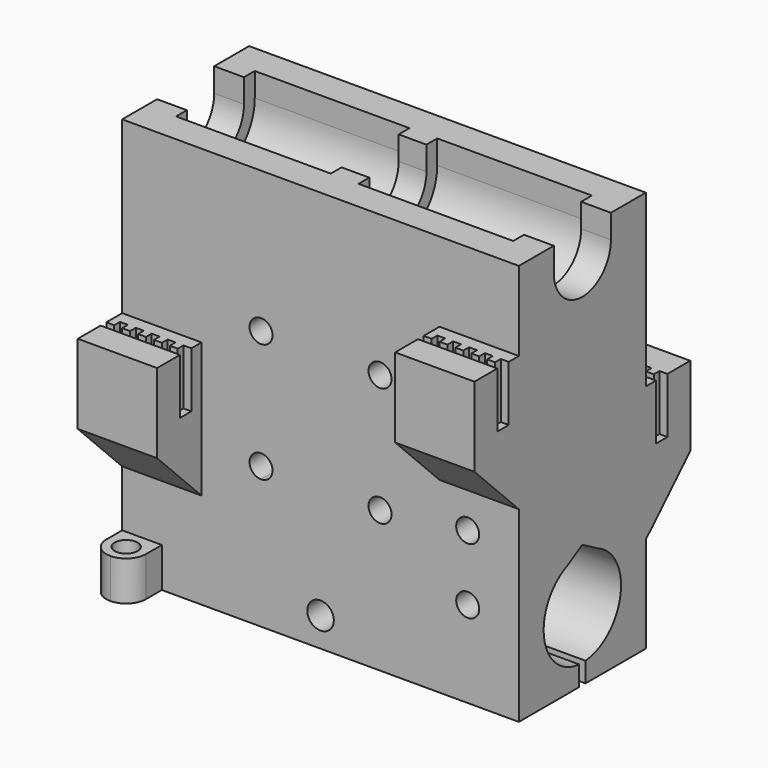
from build123d import *

# Parameters (mm, degrees)
F0_W         = 50
F0_H         = 20
F1_DEPTH     = 50.6
F3_DEPTH     = 50.001
F4_DEPTH     = 46.25
F5_DEPTH     = 26.75
F6_DEPTH     = 23.25
F7_DEPTH     = 3.75
F8_W         = 10
F8_H         = 20
F9_DEPTH     = 7
F10_T4_DEPTH = 61.4336597593
F10_T9_DEPTH = 61.4336597593
F12_DEPTH    = 7
F14_DEPTH    = 7
F15_W        = 10
F15_H        = 20
F16_DEPTH    = 7
F18_DEPTH    = 7
F20_DEPTH    = 7
F21_T4_DEPTH = 61.4336597593
F21_T9_DEPTH = 61.4336597593
F22_R        = 1.45
F22_R_2      = 1.675
F23_DEPTH    = 27.001
F24_R        = 1.45
F25_DEPTH    = 5
F26_W        = 5
F26_H        = 5
F27_DEPTH    = 5
F29_DEPTH    = 25
F30_R        = 2.49999
F32_DEPTH    = 4.5


# Not quite as in the source:
# - a fillet or chamfer that OpenCascade refuses, or shapes differently, is made with other operations: its cross-section is extruded or revolved along the edge and cut away or added
# - a fillet or chamfer is up to 0.001 mm smaller than in the source, because OpenCascade refuses the exact size


with BuildPart() as f1:
    # F0 (on Top) → F1 (new body)
    with BuildSketch(Plane.XY):
        with Locations((25, 10)):
            Rectangle(F0_W, F0_H)
    extrude(amount=F1_DEPTH)

    # F2 (on face) → F3 (cut, through all)
    with BuildSketch(Plane(origin=(0, 0, 0), x_dir=(0, -1, 0), z_dir=(-1, 0, 0))):
        with BuildLine():
            Line((-7.5528932501, 14.1876353276), (-6.3860941653, 13.5142328616))
            ThreePointArc((-6.3860941653, 13.5142328616), (-6.9508466572, 13.8832436904), (-7.5528932501, 14.1876353276))
        make_face()
        with BuildLine():
            ThreePointArc((-12.4471067499, 14.1876353276), (-13.0491533428, 13.8832436904), (-13.6139058347, 13.5142328616))
            Line((-13.6139058347, 13.5142328616), (-12.4471067499, 14.1876353276))
        make_face()
        with BuildLine():
            Line((-9.5, 0), (-9.5, 2.5205263386))
            ThreePointArc((-9.5, 2.5205263386), (-10, 2.5), (-10.5, 2.5205263386))
            Line((-10.5, 2.5205263386), (-10.5, 0))
            Line((-10.5, 0), (-10, 0))
            Line((-10, 0), (-9.5, 0))
        make_face()
        with BuildLine():
            ThreePointArc((-10.5, 2.5205263386), (-10, 2.5), (-9.5, 2.5205263386))
            Line((-9.5, 2.5205263386), (-10.5, 2.5205263386))
        make_face()
        with BuildLine():
            ThreePointArc((-10, 14.7), (-8.7499151026, 14.5705349634), (-7.5528932501, 14.1876353276))
            Line((-7.5528932501, 14.1876353276), (-10, 15.5999502167))
            Line((-10, 15.5999502167), (-10, 14.7))
        make_face()
        with BuildLine():
            ThreePointArc((-12.4471067499, 14.1876353276), (-11.2500848974, 14.5705349634), (-10, 14.7))
            Line((-10, 14.7), (-10, 15.5999502167))
            Line((-10, 15.5999502167), (-12.4471067499, 14.1876353276))
        make_face()
        with BuildLine():
            ThreePointArc((-9.5, 2.5205263386), (-5.5133531452, 4.467204336), (-3.9, 8.6))
            ThreePointArc((-3.9, 8.6), (-4.5568930935, 11.3536497969), (-6.3860941653, 13.5142328616))
            Line((-6.3860941653, 13.5142328616), (-7.5528932501, 14.1876353276))
            ThreePointArc((-7.5528932501, 14.1876353276), (-8.7499151026, 14.5705349634), (-10, 14.7))
            ThreePointArc((-10, 14.7), (-11.2500848974, 14.5705349634), (-12.4471067499, 14.1876353276))
            Line((-12.4471067499, 14.1876353276), (-13.6139058347, 13.5142328616))
            ThreePointArc((-13.6139058347, 13.5142328616), (-15.8691099055, 6.937607472), (-10.5, 2.5205263386))
            Line((-10.5, 2.5205263386), (-9.5, 2.5205263386))
        make_face()
        with BuildLine():
            Line((-5.5, 47.6), (-5.5, 50.6))
            Line((-5.5, 50.6), (-6.6458980338, 50.6))
            ThreePointArc((-6.6458980338, 50.6), (-5.7962243847, 49.205699404), (-5.5, 47.6))
        make_face()
        with BuildLine():
            Line((-13.3541019662, 50.6), (-14.5, 50.6))
            Line((-14.5, 50.6), (-14.5, 47.6))
            ThreePointArc((-14.5, 47.6), (-14.2037756153, 49.205699404), (-13.3541019662, 50.6))
        make_face()
        with BuildLine():
            ThreePointArc((-14.5, 47.6), (-10, 43.1), (-5.5, 47.6))
            ThreePointArc((-5.5, 47.6), (-5.7962243847, 49.205699404), (-6.6458980338, 50.6))
            Line((-6.6458980338, 50.6), (-13.3541019662, 50.6))
            ThreePointArc((-13.3541019662, 50.6), (-14.2037756153, 49.205699404), (-14.5, 47.6))
        make_face()
    extrude(amount=-F3_DEPTH, mode=Mode.SUBTRACT)

    # F2 (on face) → F4 (cut)
    with BuildSketch(Plane(origin=(0, 0, 0), x_dir=(0, -1, 0), z_dir=(-1, 0, 0))):
        with BuildLine():
            ThreePointArc((-16.2, 47.6), (-10, 41.4), (-3.8, 47.6))
            ThreePointArc((-3.8, 47.6), (-3.9966527372, 49.1491357726), (-4.5741360135, 50.6))
            Line((-4.5741360135, 50.6), (-5.5, 50.6))
            Line((-5.5, 50.6), (-5.5, 47.6))
            ThreePointArc((-5.5, 47.6), (-10, 43.1), (-14.5, 47.6))
            Line((-14.5, 47.6), (-14.5, 50.6))
            Line((-14.5, 50.6), (-15.4258639865, 50.6))
            ThreePointArc((-15.4258639865, 50.6), (-16.0033472628, 49.1491357726), (-16.2, 47.6))
        make_face()
        with BuildLine():
            Line((-15.4258639865, 50.6), (-16.2, 50.6))
            Line((-16.2, 50.6), (-16.2, 47.6))
            ThreePointArc((-16.2, 47.6), (-16.0033472628, 49.1491357726), (-15.4258639865, 50.6))
        make_face()
        with BuildLine():
            Line((-3.8, 47.6), (-3.8, 50.6))
            Line((-3.8, 50.6), (-4.5741360135, 50.6))
            ThreePointArc((-4.5741360135, 50.6), (-3.9966527372, 49.1491357726), (-3.8, 47.6))
        make_face()
    extrude(amount=-F4_DEPTH, mode=Mode.SUBTRACT)

    # F2 (on face) → F5 (join)
    with BuildSketch(Plane(origin=(0, 0, 0), x_dir=(0, -1, 0), z_dir=(-1, 0, 0))):
        with BuildLine():
            ThreePointArc((-16.2, 47.6), (-10, 41.4), (-3.8, 47.6))
            ThreePointArc((-3.8, 47.6), (-3.9966527372, 49.1491357726), (-4.5741360135, 50.6))
            Line((-4.5741360135, 50.6), (-5.5, 50.6))
            Line((-5.5, 50.6), (-5.5, 47.6))
            ThreePointArc((-5.5, 47.6), (-10, 43.1), (-14.5, 47.6))
            Line((-14.5, 47.6), (-14.5, 50.6))
            Line((-14.5, 50.6), (-15.4258639865, 50.6))
            ThreePointArc((-15.4258639865, 50.6), (-16.0033472628, 49.1491357726), (-16.2, 47.6))
        make_face()
        with BuildLine():
            Line((-15.4258639865, 50.6), (-16.2, 50.6))
            Line((-16.2, 50.6), (-16.2, 47.6))
            ThreePointArc((-16.2, 47.6), (-16.0033472628, 49.1491357726), (-15.4258639865, 50.6))
        make_face()
        with BuildLine():
            Line((-3.8, 47.6), (-3.8, 50.6))
            Line((-3.8, 50.6), (-4.5741360135, 50.6))
            ThreePointArc((-4.5741360135, 50.6), (-3.9966527372, 49.1491357726), (-3.8, 47.6))
        make_face()
    extrude(amount=-F5_DEPTH)

    # F2 (on face) → F6 (cut)
    with BuildSketch(Plane(origin=(0, 0, 0), x_dir=(0, -1, 0), z_dir=(-1, 0, 0))):
        with BuildLine():
            ThreePointArc((-16.2, 47.6), (-10, 41.4), (-3.8, 47.6))
            ThreePointArc((-3.8, 47.6), (-3.9966527372, 49.1491357726), (-4.5741360135, 50.6))
            Line((-4.5741360135, 50.6), (-5.5, 50.6))
            Line((-5.5, 50.6), (-5.5, 47.6))
            ThreePointArc((-5.5, 47.6), (-10, 43.1), (-14.5, 47.6))
            Line((-14.5, 47.6), (-14.5, 50.6))
            Line((-14.5, 50.6), (-15.4258639865, 50.6))
            ThreePointArc((-15.4258639865, 50.6), (-16.0033472628, 49.1491357726), (-16.2, 47.6))
        make_face()
        with BuildLine():
            Line((-15.4258639865, 50.6), (-16.2, 50.6))
            Line((-16.2, 50.6), (-16.2, 47.6))
            ThreePointArc((-16.2, 47.6), (-16.0033472628, 49.1491357726), (-15.4258639865, 50.6))
        make_face()
        with BuildLine():
            Line((-3.8, 47.6), (-3.8, 50.6))
            Line((-3.8, 50.6), (-4.5741360135, 50.6))
            ThreePointArc((-4.5741360135, 50.6), (-3.9966527372, 49.1491357726), (-3.8, 47.6))
        make_face()
    extrude(amount=-F6_DEPTH, mode=Mode.SUBTRACT)

    # F2 (on face) → F7 (join)
    with BuildSketch(Plane(origin=(0, 0, 0), x_dir=(0, -1, 0), z_dir=(-1, 0, 0))):
        with BuildLine():
            ThreePointArc((-16.2, 47.6), (-10, 41.4), (-3.8, 47.6))
            ThreePointArc((-3.8, 47.6), (-3.9966527372, 49.1491357726), (-4.5741360135, 50.6))
            Line((-4.5741360135, 50.6), (-5.5, 50.6))
            Line((-5.5, 50.6), (-5.5, 47.6))
            ThreePointArc((-5.5, 47.6), (-10, 43.1), (-14.5, 47.6))
            Line((-14.5, 47.6), (-14.5, 50.6))
            Line((-14.5, 50.6), (-15.4258639865, 50.6))
            ThreePointArc((-15.4258639865, 50.6), (-16.0033472628, 49.1491357726), (-16.2, 47.6))
        make_face()
        with BuildLine():
            Line((-15.4258639865, 50.6), (-16.2, 50.6))
            Line((-16.2, 50.6), (-16.2, 47.6))
            ThreePointArc((-16.2, 47.6), (-16.0033472628, 49.1491357726), (-15.4258639865, 50.6))
        make_face()
        with BuildLine():
            Line((-3.8, 47.6), (-3.8, 50.6))
            Line((-3.8, 50.6), (-4.5741360135, 50.6))
            ThreePointArc((-4.5741360135, 50.6), (-3.9966527372, 49.1491357726), (-3.8, 47.6))
        make_face()
    extrude(amount=-F7_DEPTH)

    # F8 (on face) → F9 (join)
    with BuildSketch(Plane.XZ):
        with Locations((5, 19.1)):
            Rectangle(F8_W, F8_H)
        with Locations((45, 30.6)):
            Rectangle(F8_W, F8_H)
    extrude(amount=F9_DEPTH)

    # F10: chamfer of 10 on 2 edges, made by hand


with BuildPart() as f10_tool2:
    # F10_s3 → F10_t4 (new body)
    with BuildSketch(Plane.YZ.offset(-25.7168298797)):
        Polygon((3, 9.1), (-7, 19.1), (-7, 9.1), align=None)
    extrude(amount=F10_T4_DEPTH)

    split(bisect_by=Plane.XZ, keep=Keep.TOP)


with BuildPart() as f1_1:
    add(f1.part)

    # F10_t1: cut F10_tool2
    add(f10_tool2.part, mode=Mode.SUBTRACT)


with BuildPart() as f10_tool7:
    # F10_s8 → F10_t9 (new body)
    with BuildSketch(Plane.YZ.offset(14.2831701203)):
        Polygon((3, 20.6), (-7, 30.6), (-7, 20.6), align=None)
    extrude(amount=F10_T9_DEPTH)

    split(bisect_by=Plane.XZ, keep=Keep.TOP)


with BuildPart() as f1_2:
    add(f1_1.part)

    # F10_t6: cut F10_tool7
    add(f10_tool7.part, mode=Mode.SUBTRACT)

    # F11 (on face) → F12 (cut)
    with BuildSketch(Plane.XY.offset(29.1)):
        Polygon((0, -2.5), (0, -3.4), (10, -3.4), (10, -2.5), (10, -1.6), (9, -1.6), (9, -2.5), (8, -2.5), (8, -1.6), (7, -1.6), (7, -2.5), (6, -2.5), (6, -1.6), (5.2958247252, -1.6), (5, -1.6), (5, -2.5), (4, -2.5), (4, -1.6), (3, -1.6), (3, -2.5), (2, -2.5), (2, -1.6), (1, -1.6), (1, -2.5), align=None)
    extrude(amount=-F12_DEPTH, mode=Mode.SUBTRACT)

    # F13 (on face) → F14 (cut)
    with BuildSketch(Plane.XY.offset(40.6)):
        Polygon((40, -2.5), (40, -3.4), (50, -3.4), (50, -2.5), (50, -1.6), (49, -1.6), (49, -2.5), (48, -2.5), (48, -1.6), (47, -1.6), (47, -2.5), (46, -2.5), (46, -1.6), (45.2349036932, -1.6), (45, -1.6), (45, -2.5), (44, -2.5), (44, -1.6), (43, -1.6), (43, -2.5), (42, -2.5), (42, -1.6), (41, -1.6), (41, -2.5), align=None)
    extrude(amount=-F14_DEPTH, mode=Mode.SUBTRACT)

    # F15 (on face) → F16 (join)
    with BuildSketch(Plane(origin=(0, 20, 0), x_dir=(-1, 0, 0), z_dir=(0, 1, 0))):
        with Locations((-45, 19.1)):
            Rectangle(F15_W, F15_H)
        with Locations((-5, 30.6)):
            Rectangle(F15_W, F15_H)
    extrude(amount=F16_DEPTH)

    # F17 (on face) → F18 (cut)
    with BuildSketch(Plane.XY.offset(29.1)):
        Polygon((40, 22.5), (40, 21.6), (45, 21.6), (50, 21.6), (50, 22.5), (50, 23.4), (49, 23.4), (49, 22.5), (48, 22.5), (48, 23.4), (47, 23.4), (47, 22.5), (46, 22.5), (46, 23.4), (45, 23.4), (45, 22.5), (44, 22.5), (44, 23.4), (43, 23.4), (43, 22.5), (42, 22.5), (42, 23.4), (41, 23.4), (41, 22.5), align=None)
    extrude(amount=-F18_DEPTH, mode=Mode.SUBTRACT)

    # F19 (on face) → F20 (cut)
    with BuildSketch(Plane.XY.offset(40.6)):
        Polygon((7, 22.5), (6, 22.5), (6, 23.4), (5, 23.4), (5, 22.5), (4, 22.5), (4, 23.4), (3, 23.4), (3, 22.5), (2, 22.5), (2, 23.4), (1, 23.4), (1, 22.5), (0, 22.5), (0, 21.6), (5, 21.6), (10, 21.6), (10, 22.5), (10, 23.4), (9, 23.4), (9, 22.5), (8, 22.5), (8, 23.4), (7, 23.4), align=None)
    extrude(amount=-F20_DEPTH, mode=Mode.SUBTRACT)

    # F21: chamfer of 10 on 2 edges, made by hand


with BuildPart() as f21_tool2:
    # F21_s3 → F21_t4 (new body)
    with BuildSketch(Plane.YZ.offset(35.7168298797)):
        Polygon((27, 30.6), (17, 20.6), (27, 20.6), align=None)
    extrude(amount=-F21_T4_DEPTH)

    split(bisect_by=Plane.XZ.offset(-20), keep=Keep.BOTTOM)


with BuildPart() as f1_3:
    add(f1_2.part)

    # F21_t1: cut F21_tool2
    add(f21_tool2.part, mode=Mode.SUBTRACT)


with BuildPart() as f21_tool7:
    # F21_s8 → F21_t9 (new body)
    with BuildSketch(Plane.YZ.offset(75.7168298797)):
        Polygon((17, 9.1), (27, 19.1), (27, 9.1), align=None)
    extrude(amount=-F21_T9_DEPTH)

    split(bisect_by=Plane.XZ.offset(-20), keep=Keep.BOTTOM)


with BuildPart() as f1_4:
    add(f1_3.part)

    # F21_t6: cut F21_tool7
    add(f21_tool7.part, mode=Mode.SUBTRACT)

    # F22 (on face) → F23 (cut, through all)
    with BuildSketch(Plane.XZ):
        with BuildLine():
            ThreePointArc((16.05, 32.8), (17.5, 31.35), (18.95, 32.8))
            ThreePointArc((18.95, 32.8), (17.5, 34.25), (16.05, 32.8))
        make_face()
        with BuildLine():
            ThreePointArc((32.5, 34.25), (31.4746951673, 31.7746951673), (33.95, 32.8))
            ThreePointArc((33.95, 32.8), (33.5253048327, 33.8253048327), (32.5, 34.25))
        make_face()
        with BuildLine():
            ThreePointArc((17.5, 16.35), (18.5253048327, 16.7746951673), (18.95, 17.8))
            ThreePointArc((18.95, 17.8), (16.4746951673, 18.8253048327), (17.5, 16.35))
        make_face()
        with Locations((32.5, 17.8)):
            Circle(F22_R)
        with Locations((25, 3.675)):
            Circle(F22_R_2)
        with BuildLine():
            ThreePointArc((33.95, 32.8), (33.5253048327, 33.8253048327), (32.5, 34.25))
            ThreePointArc((32.5, 34.25), (31.4746951673, 31.7746951673), (33.95, 32.8))
        make_face()
        with BuildLine():
            ThreePointArc((18.95, 17.8), (16.4746951673, 18.8253048327), (17.5, 16.35))
            ThreePointArc((17.5, 16.35), (18.5253048327, 16.7746951673), (18.95, 17.8))
        make_face()
    extrude(amount=-F23_DEPTH, mode=Mode.SUBTRACT)

    # F24 (on face) → F25 (cut)
    with BuildSketch(Plane.XZ):
        with Locations((43.55, 19.15)):
            Circle(F24_R)
        with Locations((43.55, 10.9)):
            Circle(F24_R)
    extrude(amount=-F25_DEPTH, mode=Mode.SUBTRACT)

    # F26 (on face) → F27 (join)
    with BuildSketch(Plane.XZ):
        with Locations((2.5, 2.5)):
            Rectangle(F26_W, F26_H)
    extrude(amount=F27_DEPTH)

    # F28 (on face) → F29 (cut)
    with BuildSketch(Plane.XY.offset(5)):
        with BuildLine():
            Line((1.05, -2.5), (3.95, -2.5))
            ThreePointArc((3.95, -2.5), (2.5, -1.05), (1.05, -2.5))
        make_face()
        with BuildLine():
            ThreePointArc((1.05, -2.5), (2.5, -3.95), (3.95, -2.5))
            Line((3.95, -2.5), (1.05, -2.5))
        make_face()
    extrude(amount=-F29_DEPTH, mode=Mode.SUBTRACT)

    # F30 (radius 2.5 in the source; OpenCascade refuses exactly that, so slightly less here)
    f30_edges = [f1_4.edges().sort_by_distance(p)[0] for p in [
        (0, -5, 2.5),
        (5, -5, 2.5),
    ]]
    fillet(f30_edges, radius=F30_R)

    # F31 (on face) → F32 (cut)
    with BuildSketch(Plane(origin=(0, 0, 0), x_dir=(1, 0, 0), z_dir=(0, 0, -1))):
        with BuildLine():
            ThreePointArc((3.95, -16.5), (3.5253048327, -15.4746951673), (2.5, -15.05))
            ThreePointArc((2.5, -15.05), (1.4746951673, -17.5253048327), (3.95, -16.5))
        make_face()
    extrude(amount=-F32_DEPTH, mode=Mode.SUBTRACT)


solid = f1_4.part
